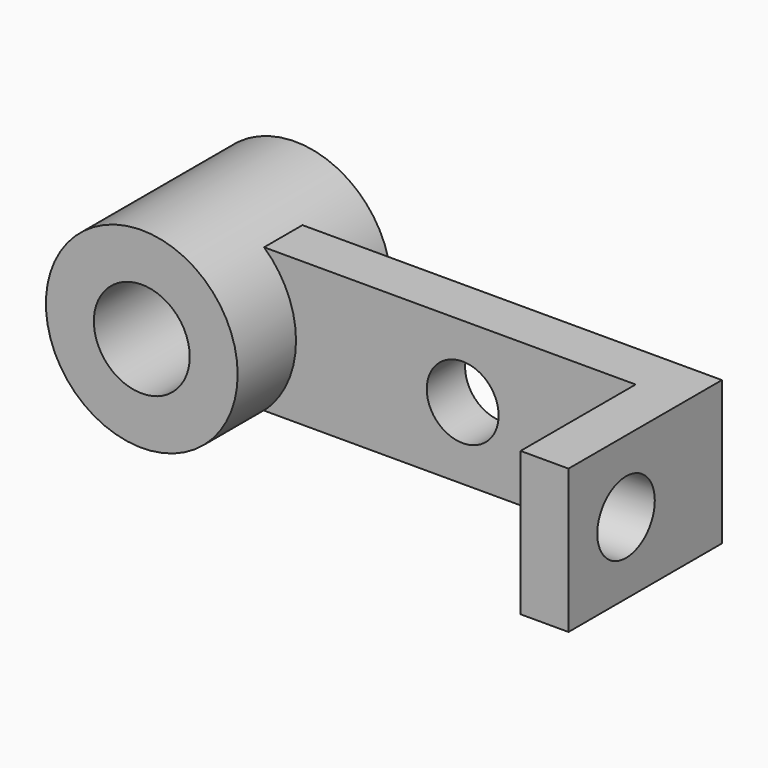
from build123d import *

# Parameters (mm, degrees)
F0_R      = 20
F0_R_2    = 10
F1_DEPTH  = 40
F4_DEPTH  = 40
F5_W      = 77.4922952824
F5_H      = 30
F6_DEPTH  = 35.1464343736
F7_R      = 7.5
F8_DEPTH  = 40.001
F9_R      = 7.5
F10_DEPTH = 121.0079549157


with BuildPart() as f1:
    # F0 (on Front) → F1 (new body)
    with BuildSketch(Plane.XZ):
        with Locations((0.0621909407, 19.8545656264)):
            Circle(F0_R)
        with Locations((0.0621909407, 19.8545656264)):
            Circle(F0_R_2, mode=Mode.SUBTRACT)
    extrude(amount=F1_DEPTH)


with BuildPart() as f4:
    # F3 (on offset) → F4 (new body)
    with BuildSketch(Plane(origin=(0, -15, 0), x_dir=(-1, 0, 0), z_dir=(0, 1, 0))):
        with BuildLine():
            Line((-101.0691458563, 35), (-101.0691458563, 20))
            Line((-101.0691458563, 20), (-101.0691458563, 5))
            Line((-101.0691458563, 5), (-13.576850574, 5))
            ThreePointArc((-13.576850574, 5), (-20.231927034, 20), (-13.576850574, 35))
            Line((-13.576850574, 35), (-101.0691458563, 35))
        make_face()
    extrude(amount=-F4_DEPTH)

    # F5 (on face) → F6 (cut, through all)
    with BuildSketch(Plane.XY.offset(35)):
        with Locations((52.3229982152, -40)):
            Rectangle(F5_W, F5_H)
    extrude(amount=-F6_DEPTH, mode=Mode.SUBTRACT)

    # F7 (on face) → F8 (cut, through all)
    with BuildSketch(Plane(origin=(0, -15, 0), x_dir=(-1, 0, 0), z_dir=(0, 1, 0))):
        with Locations((-55, 20)):
            Circle(F7_R)
    extrude(amount=-F8_DEPTH, mode=Mode.SUBTRACT)

    # F9 (on face) → F10 (cut, through all)
    with BuildSketch(Plane.YZ.offset(101.0691458563)):
        with Locations((-40, 20)):
            Circle(F9_R)
    extrude(amount=-F10_DEPTH, mode=Mode.SUBTRACT)


solid = Compound([f1.part, f4.part])
